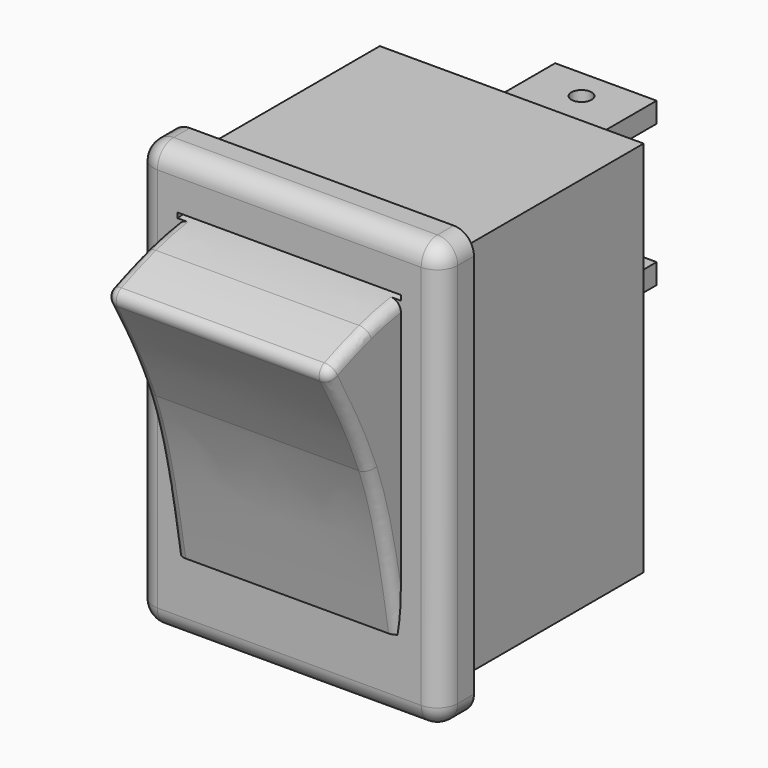
from build123d import *

# Parameters (mm, degrees)
F0_W      = 13
F0_H      = 18.6
F1_DEPTH  = 11.7
F2_W      = 15
F2_H      = 21
F3_DEPTH  = 2
F5_START  = 1
F5_DEPTH  = 11
F6_START  = 1
F6_DEPTH  = 11
F7_R      = 1
F8_R      = 0.5
F9_W      = 5
F9_H      = 1
F10_DEPTH = 6.3
F11_SIZE  = 0.49999
F12_R     = 0.5
F13_DEPTH = 25


# Not quite as in the source:
# - a fillet or chamfer is up to 0.001 mm smaller than in the source, because OpenCascade refuses the exact size


with BuildPart() as f1:
    # F0 (on Front) → F1 (new body)
    with BuildSketch(Plane.XZ):
        with Locations((6.5, 9.3)):
            Rectangle(F0_W, F0_H)
    extrude(amount=-F1_DEPTH)

    # F2 (on Front) → F3 (join)
    with BuildSketch(Plane.XZ):
        with Locations((6.5, 9.3)):
            Rectangle(F2_W, F2_H)
    extrude(amount=F3_DEPTH)

    # F4 (on Right) → F5 (cut)
    with BuildSketch(Plane.YZ.offset(F5_START)):
        with BuildLine():
            add(Edge.make_bspline(
                [(0, 17.2755792737), (-1.1526457271, 17.1501791024), (-2.4983857291, 17.0037715611), (-3.7827872231, 16.6499606711), (-3.9660306647, 16.5956447667)],
                knots=[0, 0, 0, 0, 0.5019383156, 0.586024356, 0.586024356, 0.586024356, 0.586024356], degree=3))
            Line((0, 17.2755792737), (-3.9660306647, 17.2755792737))
            Line((-3.9660306647, 17.2755792737), (-3.9660306647, 16.5956447667))
        make_face()
        with BuildLine():
            Line((-3.9660306647, 2.481617732), (-2.1293810569, 2.481617732))
            add(Edge.make_bspline(
                [(-3.9660306647, 10.2878685019), (-3.8996200875, 10.1138282619), (-3.0167436481, 7.7059620865), (-2.5562801998, 4.9949850403), (-2.1293810569, 2.481617732)],
                knots=[0.4423976039, 0.4423976039, 0.4423976039, 0.4423976039, 0.4830426044, 1, 1, 1, 1], degree=3))
            Line((-3.9660306647, 10.2878685019), (-3.9660306647, 2.481617732))
        make_face()
        with BuildLine():
            add(Edge.make_bspline(
                [(-3.9660306647, 10.2878685019), (-3.8996200875, 10.1138282619), (-3.0167436481, 7.7059620865), (-2.5562801998, 4.9949850403), (-2.1293810569, 2.481617732)],
                knots=[0.4423976039, 0.4423976039, 0.4423976039, 0.4423976039, 0.4830426044, 1, 1, 1, 1], degree=3))
            Line((-2.1293810569, 2.481617732), (0, 2.481617732))
            Line((0, 2.481617732), (0, 17.2755792737))
            add(Edge.make_bspline(
                [(0, 17.2755792737), (-1.1526457271, 17.1501791024), (-2.4983857291, 17.0037715611), (-3.7827872231, 16.6499606711), (-3.9660306647, 16.5956447667)],
                knots=[0, 0, 0, 0, 0.5019383156, 0.586024356, 0.586024356, 0.586024356, 0.586024356], degree=3))
            Line((-3.9660306647, 16.5956447667), (-3.9660306647, 10.2878685019))
        make_face()
    extrude(amount=F5_DEPTH, mode=Mode.SUBTRACT)

    # F4 (on Right) → F6 (join)
    with BuildSketch(Plane.YZ.offset(F6_START)):
        with BuildLine():
            add(Edge.make_bspline(
                [(-3.9660306647, 10.2878685019), (-3.8996200875, 10.1138282619), (-3.0167436481, 7.7059620865), (-2.5562801998, 4.9949850403), (-2.1293810569, 2.481617732)],
                knots=[0.4423976039, 0.4423976039, 0.4423976039, 0.4423976039, 0.4830426044, 1, 1, 1, 1], degree=3))
            Line((-2.1293810569, 2.481617732), (0, 2.481617732))
            Line((0, 2.481617732), (0, 17.2755792737))
            add(Edge.make_bspline(
                [(0, 17.2755792737), (-1.1526457271, 17.1501791024), (-2.4983857291, 17.0037715611), (-3.7827872231, 16.6499606711), (-3.9660306647, 16.5956447667)],
                knots=[0, 0, 0, 0, 0.5019383156, 0.586024356, 0.586024356, 0.586024356, 0.586024356], degree=3))
            Line((-3.9660306647, 16.5956447667), (-3.9660306647, 10.2878685019))
        make_face()
        with BuildLine():
            add(Edge.make_bspline(
                [(-6.621601202, 15.6213638948), (-5.6552365252, 13.9017804778), (-4.6888718484, 12.1821970608), (-3.9660306647, 10.2878685019)],
                knots=[0, 0, 0, 0, 0.4423976039, 0.4423976039, 0.4423976039, 0.4423976039], degree=3))
            Line((-3.9660306647, 10.2878685019), (-3.9660306647, 16.5956447667))
            add(Edge.make_bspline(
                [(-3.9660306647, 16.5956447667), (-4.8681818595, 16.3282346066), (-5.7448915308, 15.9747992507), (-6.621601202, 15.6213638948)],
                knots=[0.586024356, 0.586024356, 0.586024356, 0.586024356, 1, 1, 1, 1], degree=3))
        make_face()
    extrude(amount=F6_DEPTH)

    # F7
    f7_edges = [f1.edges().sort_by_distance(p)[0] for p in [
        (14, -1, -1.2),
        (-1, -1, -1.2),
        (-1, -1, 19.8),
        (14, -1, 19.8),
        (14, -2, 9.3),
        (6.5, -2, -1.2),
        (-1, -2, 9.3),
        (6.5, -2, 19.8),
    ]]
    fillet(f7_edges, radius=F7_R)

    # F8
    f8_edges = [f1.edges().sort_by_distance(p)[0] for p in [
        (1, -4.35533, 16.47468),
        (1, -3.6216, 9.312473),
        (6.5, -6.621601, 15.621364),
        (12, -3.6216, 9.312473),
        (12, -4.35533, 16.47468),
    ]]
    fillet(f8_edges, radius=F8_R)

    # F9 (on face) → F10 (join)
    with BuildSketch(Plane(origin=(0, 11.7, 0), x_dir=(-1, 0, 0), z_dir=(0, 1, 0))):
        with Locations((-6.5, 9.3)):
            Rectangle(F9_W, F9_H)
        with Locations((-6.5, 16.3)):
            Rectangle(F9_W, F9_H)
    extrude(amount=F10_DEPTH)

    # F11 (size 0.5 in the source; OpenCascade refuses exactly that, so slightly less here)
    f11_edges = [f1.edges().sort_by_distance(p)[0] for p in [
        (4, 18, 16.3),
        (9, 18, 16.3),
        (4, 18, 9.3),
        (9, 18, 9.3),
        (6.5, 18, 16.8),
        (6.5, 18, 15.8),
        (6.5, 18, 9.8),
        (6.5, 18, 8.8),
    ]]
    chamfer(f11_edges, length=F11_SIZE)

    # F12 (on face) → F13 (cut)
    with BuildSketch(Plane.XY.offset(16.8)):
        with Locations((6.5, 16)):
            Circle(F12_R)
    extrude(amount=-F13_DEPTH, mode=Mode.SUBTRACT)


solid = f1.part
